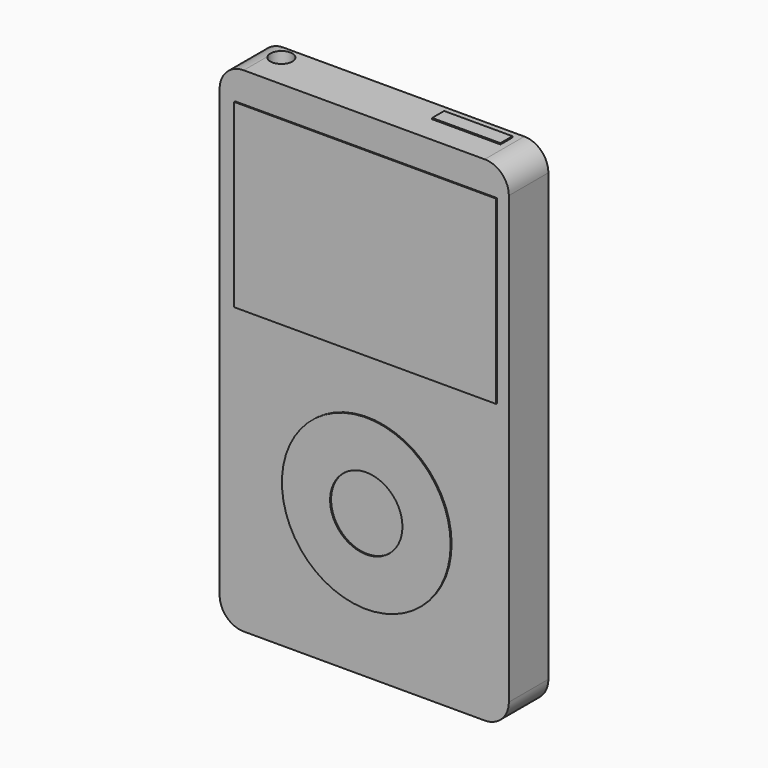
from build123d import *

# Parameters (mm, degrees)
F0_W         = 60.96
F0_H         = 104.14
F1_DEPTH     = 10.414
F3_R         = 17.78
F3_R_2       = 7.62
F4_DEPTH     = 0.254
F2_W         = 55.1793798804
F2_H         = 38.1
F5_DEPTH     = 0.254
F6_R         = 2.3165887379
F7_DEPTH     = 25.4
F8_W         = 14.3902888522
F8_H         = 3.1658638036
F9_DEPTH     = 0.254
F10_W        = 20.8778993692
F10_H        = 2.1391292103
F11_DEPTH    = 25.4
F12_R        = 5.08
F13_T1_DEPTH = 35.814
F14_R        = 5.08
F15_R        = 5.08


# Not quite as in the source:
# - a fillet or chamfer that OpenCascade refuses, or shapes differently, is made with other operations: its cross-section is extruded or revolved along the edge and cut away or added


with BuildPart() as f1:
    # F0 (on Front) → F1 (new body)
    with BuildSketch(Plane.XZ):
        with Locations((-7.5916079104, 5.2405595779)):
            Rectangle(F0_W, F0_H)
    extrude(amount=F1_DEPTH)

    # F3 (on face) → F4 (join)
    with BuildSketch(Plane.XZ.offset(10.414)):
        with Locations((-6.9598197006, -16.3494404221)):
            Circle(F3_R)
        with Locations((-6.9598197006, -16.3494404221)):
            Circle(F3_R_2, mode=Mode.SUBTRACT)
    extrude(amount=F4_DEPTH)

    # F2 (on face) → F5 (join)
    with BuildSketch(Plane.XZ.offset(10.414)):
        with Locations((-7.2018355131, 31.9105595779)):
            Rectangle(F2_W, F2_H)
    extrude(amount=F5_DEPTH)

    # F6 (on face) → F7 (cut)
    with BuildSketch(Plane.XY.offset(57.3105595779)):
        with Locations((-31.0040302575, -2.9813330621)):
            Circle(F6_R)
    extrude(amount=-F7_DEPTH, mode=Mode.SUBTRACT)

    # F8 (on face) → F9 (join)
    with BuildSketch(Plane.XY.offset(57.3105595779)):
        with Locations((9.3301092274, -3.0921686557)):
            Rectangle(F8_W, F8_H)
    extrude(amount=F9_DEPTH)

    # F10 (on face) → F11 (cut)
    with BuildSketch(Plane(origin=(0, 0, -46.8294404221), x_dir=(1, 0, 0), z_dir=(0, 0, -1))):
        with Locations((-6.7444174783, 3.3060612623)):
            Rectangle(F10_W, F10_H)
    extrude(amount=-F11_DEPTH, mode=Mode.SUBTRACT)

    # F12
    f12_edges = [f1.edges().sort_by_distance(p)[0] for p in [
        (-38.071608, -5.207, -46.82944),
    ]]
    fillet(f12_edges, radius=F12_R)

    # F13: fillet of radius 5.08 on 1 edges, made by hand

    # F13_s2 → F13_t1 (cut)
    with BuildSketch(Plane.XZ.offset(-12.7)):
        with BuildLine():
            ThreePointArc((-38.0716079104, 52.2305595779), (-36.5837103588, 55.8226620264), (-32.9916079104, 57.3105595779))
            Line((-32.9916079104, 57.3105595779), (-38.0716079104, 57.3105595779))
            Line((-38.0716079104, 57.3105595779), (-38.0716079104, 52.2305595779))
        make_face()
    extrude(amount=F13_T1_DEPTH, mode=Mode.SUBTRACT)

    # F14
    f14_edges = [f1.edges().sort_by_distance(p)[0] for p in [
        (22.888392, -5.207, -46.82944),
    ]]
    fillet(f14_edges, radius=F14_R)

    # F15
    f15_edges = [f1.edges().sort_by_distance(p)[0] for p in [
        (22.888392, -5.207, 57.31056),
    ]]
    fillet(f15_edges, radius=F15_R)


solid = f1.part
